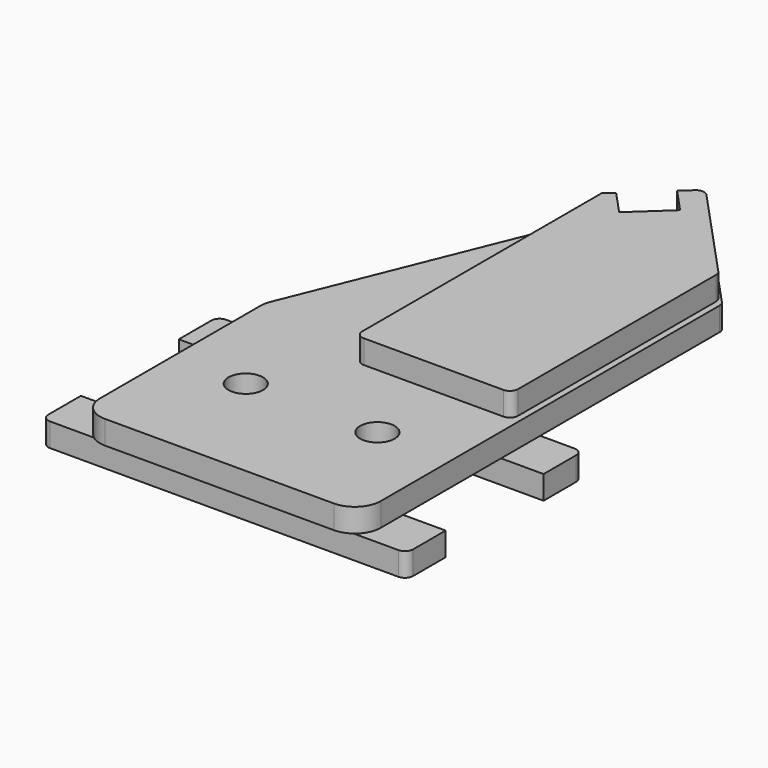
from build123d import *

# Parameters (mm, degrees)
F0_R     = 10.5
F1_DEPTH = 14.2875
F2_W     = 170
F2_H     = 29.6946875751
F3_DEPTH = 14.2875
F5_DEPTH = 14.2875


# Not quite as in the source:
# - a length typed as a fraction of an inch, garbled in the dataset ("3 / 203.2 mm" for 3/8 in), is restored
# - a feature names something its author has since deleted; it is built from what else it names


with BuildPart() as f1:
    # F0 (on Top) → F1 (new body)
    with BuildSketch(Plane.XY):
        with BuildLine():
            ThreePointArc((-84.5842045546, -55), (-80.1908062724, -65.6066017178), (-69.5842045546, -70))
            Line((-69.5842045546, -70), (69.5842045546, -70))
            ThreePointArc((69.5842045546, -70), (80.7788298305, -65.363034385), (85.4157954454, -54.1684091091))
            Line((85.4157954454, -54.1684091091), (85.4157954454, 203.1919921827))
            ThreePointArc((85.4157954454, 203.1919921827), (85.0717839963, 205.0145647093), (84.0870871996, 206.5863429094))
            Line((84.0870871996, 206.5863429094), (27.5340619023, 267.7534620916))
            ThreePointArc((27.5340619023, 267.7534620916), (24.0585970267, 269.3552750765), (20.4684194215, 268.030403119))
            Line((20.4684194215, 268.030403119), (13.1258359132, 261.2417016656))
            Line((13.1258359132, 261.2417016656), (26.70323882, 246.556534649))
            Line((26.70323882, 246.556534649), (16.0564927329, 236.7129175415))
            Line((16.0564927329, 236.7129175415), (5.4097466459, 226.8693004341))
            Line((5.4097466459, 226.8693004341), (-8.1676562609, 241.5544674507))
            Line((-8.1676562609, 241.5544674507), (-18.3614984488, 232.1295897903))
            ThreePointArc((-18.3614984488, 232.1295897903), (-19.0801780579, 231.3013565049), (-19.6010257192, 230.336375433))
            Line((-19.6010257192, 230.336375433), (-83.4858385457, 72.7100555545))
            ThreePointArc((-83.4858385457, 72.7100555545), (-84.3070526124, 69.9459705844), (-84.5842045546, 67.0758233641))
            Line((-84.5842045546, 67.0758233641), (-84.5842045546, -55))
        make_face()
        with Locations((-40, 0)):
            Circle(F0_R, mode=Mode.SUBTRACT)
        with Locations((40, 0)):
            Circle(F0_R, mode=Mode.SUBTRACT)
    extrude(amount=F1_DEPTH)

    # F2 (on face) → F3 (join)
    with BuildSketch(Plane(origin=(0, 0, 0), x_dir=(1, 0, 0), z_dir=(0, 0, -1))):
        with BuildLine():
            ThreePointArc((-110.4471534491, -61.8855160475), (-108.982687355, -65.4210499534), (-105.4471534491, -66.8855160475))
            Line((-105.4471534491, -66.8855160475), (-84.5842045546, -66.8855160475))
            Line((-84.5842045546, -66.8855160475), (-84.5842045546, -37.1908284724))
            Line((-84.5842045546, -37.1908284724), (-110.4471534491, -37.1908284724))
            Line((-110.4471534491, -37.1908284724), (-110.4471534491, -61.8855160475))
        make_face()
        with Locations((0.4157954454, -52.0381722599)):
            Rectangle(F2_W, F2_H)
        with BuildLine():
            Line((85.4157954454, -37.1908284724), (85.4157954454, -66.8855160475))
            Line((85.4157954454, -66.8855160475), (106.2211793661, -66.8855160475))
            ThreePointArc((106.2211793661, -66.8855160475), (109.756713272, -65.4210499534), (111.2211793661, -61.8855160475))
            Line((111.2211793661, -61.8855160475), (111.2211793661, -37.1908284724))
            Line((111.2211793661, -37.1908284724), (85.4157954454, -37.1908284724))
        make_face()
        with BuildLine():
            Line((-84.5842045546, 55), (-84.5842045546, 37.1908284724))
            Line((-84.5842045546, 37.1908284724), (85.4157954454, 37.1908284724))
            Line((85.4157954454, 37.1908284724), (85.4157954454, 54.1684091091))
            ThreePointArc((85.4157954454, 54.1684091091), (83.7249684911, 61.287261926), (79.0136510523, 66.8855160475))
            Line((79.0136510523, 66.8855160475), (-78.7348607215, 66.8855160475))
            ThreePointArc((-78.7348607215, 66.8855160475), (-83.0426562208, 61.623449158), (-84.5842045546, 55))
        make_face()
        with BuildLine():
            Line((-110.4471534491, 37.1908284724), (-84.5842045546, 37.1908284724))
            Line((-84.5842045546, 37.1908284724), (-84.5842045546, 55))
            ThreePointArc((-84.5842045546, 55), (-83.0426562208, 61.623449158), (-78.7348607215, 66.8855160475))
            Line((-78.7348607215, 66.8855160475), (-105.4471534491, 66.8855160475))
            ThreePointArc((-105.4471534491, 66.8855160475), (-108.982687355, 65.4210499534), (-110.4471534491, 61.8855160475))
            Line((-110.4471534491, 61.8855160475), (-110.4471534491, 37.1908284724))
        make_face()
        with BuildLine():
            Line((85.4157954454, 54.1684091091), (85.4157954454, 37.1908284724))
            Line((85.4157954454, 37.1908284724), (111.2211793661, 37.1908284724))
            Line((111.2211793661, 37.1908284724), (111.2211793661, 61.8855160475))
            ThreePointArc((111.2211793661, 61.8855160475), (109.756713272, 65.4210499534), (106.2211793661, 66.8855160475))
            Line((106.2211793661, 66.8855160475), (79.0136510523, 66.8855160475))
            ThreePointArc((79.0136510523, 66.8855160475), (83.7249684911, 61.287261926), (85.4157954454, 54.1684091091))
        make_face()
    extrude(amount=F3_DEPTH)

    # F4 (on face) → F5 (join)
    with BuildSketch(Plane.XY.offset(14.2875)):
        with BuildLine():
            Line((-8.2645773549, 49.9606142757), (76.5538805598, 49.9606142757))
            ThreePointArc((76.5538805598, 49.9606142757), (80.0894144658, 51.4250803698), (81.5538805598, 54.9606142757))
            Line((81.5538805598, 54.9606142757), (81.5538805598, 205.2832095857))
            ThreePointArc((81.5538805598, 205.2832095857), (81.2098691107, 207.1057821123), (80.225172314, 208.6775603124))
            Line((80.225172314, 208.6775603124), (26.4943680898, 266.7921967701))
            ThreePointArc((26.4943680898, 266.7921967701), (23.0189032141, 268.3940097551), (19.4287256089, 267.0691377976))
            Line((19.4287256089, 267.0691377976), (13.1258359132, 261.2417016656))
            Line((13.1258359132, 261.2417016656), (26.70323882, 246.556534649))
            Line((26.70323882, 246.556534649), (5.4097466459, 226.8693004341))
            Line((5.4097466459, 226.8693004341), (-8.1676562609, 241.5544674507))
            Line((-8.1676562609, 241.5544674507), (-13.2645773549, 236.8420286205))
            Line((-13.2645773549, 236.8420286205), (-13.2645773549, 54.9606142757))
            ThreePointArc((-13.2645773549, 54.9606142757), (-11.8001112608, 51.4250803698), (-8.2645773549, 49.9606142757))
        make_face()
    extrude(amount=F5_DEPTH)


solid = f1.part
